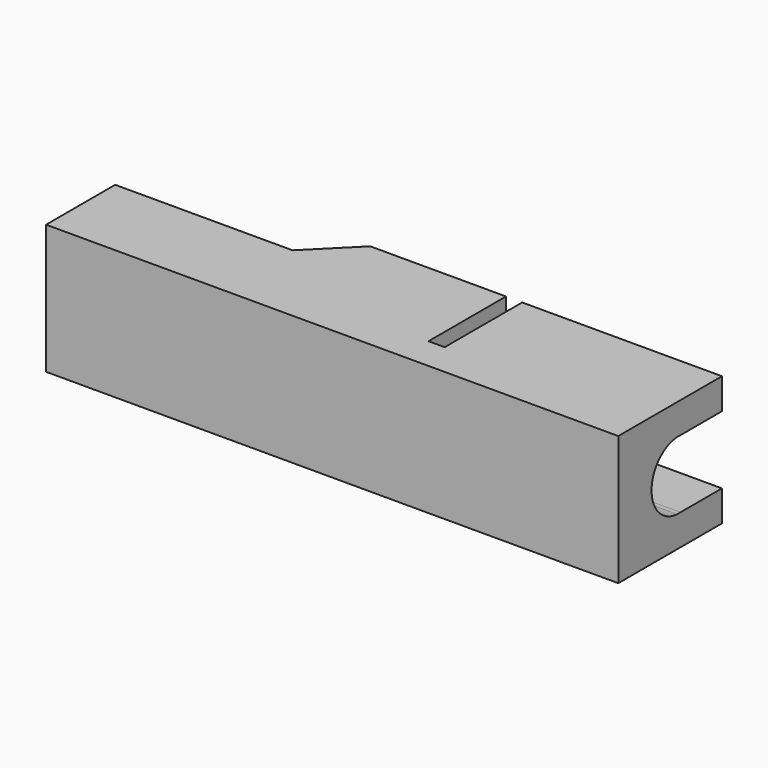
from build123d import *

# Parameters (mm, degrees)
F0_W      = 93
F0_H      = 10
F1_DEPTH  = 12
F3_DEPTH  = 90
F5_W      = 8.9714768017
F5_H      = 12
F6_DEPTH  = 1.5
F7_DEPTH  = 2
F8_DEPTH  = 40
F9_W      = 20.4241964966
F9_H      = 12
F10_DEPTH = 4
F11_SIZE  = 3.99999


# Not quite as in the source:
# - a fillet or chamfer is up to 0.001 mm smaller than in the source, because OpenCascade refuses the exact size


with BuildPart() as f1:
    # F0 (on Top) → F1 (new body)
    with BuildSketch(Plane.XY):
        with Locations((46.5, 5)):
            Rectangle(F0_W, F0_H)
    extrude(amount=F1_DEPTH)

    # F2 (on face) → F3 (cut)
    with BuildSketch(Plane.YZ.offset(93)):
        with BuildLine():
            Line((4.8075824627, 6), (4.8075824627, 9.1441176014))
            ThreePointArc((4.8075824627, 9.1441176014), (1.85, 6), (4.8075824627, 2.8558823986))
            Line((4.8075824627, 2.8558823986), (4.8075824627, 6))
        make_face()
        with BuildLine():
            ThreePointArc((5.1924175373, 9.1441176014), (5, 9.15), (4.8075824627, 9.1441176014))
            Line((4.8075824627, 9.1441176014), (5.1924175373, 9.1441176014))
        make_face()
        with BuildLine():
            Line((5.1924175373, 9.1441176014), (4.8075824627, 9.1441176014))
            Line((4.8075824627, 9.1441176014), (4.8075824627, 6))
            Line((4.8075824627, 6), (8.15, 6))
            ThreePointArc((8.15, 6), (7.2944079021, 8.1582845917), (5.1924175373, 9.1441176014))
        make_face()
        with BuildLine():
            Line((5.1924175373, 2.8558823986), (4.8075824627, 2.8558823986))
            ThreePointArc((4.8075824627, 2.8558823986), (5, 2.85), (5.1924175373, 2.8558823986))
        make_face()
        with BuildLine():
            Line((4.8075824627, 6), (4.8075824627, 2.8558823986))
            Line((4.8075824627, 2.8558823986), (5.1924175373, 2.8558823986))
            ThreePointArc((5.1924175373, 2.8558823986), (7.2944079021, 3.8417154083), (8.15, 6))
            Line((8.15, 6), (4.8075824627, 6))
        make_face()
        with BuildLine():
            Line((10, 9.1441176014), (5.1924175373, 9.1441176014))
            ThreePointArc((5.1924175373, 9.1441176014), (7.2944079021, 8.1582845917), (8.15, 6))
            Line((8.15, 6), (10, 6))
            Line((10, 6), (10, 9.1441176014))
        make_face()
        with BuildLine():
            ThreePointArc((8.15, 6), (7.2944079021, 3.8417154083), (5.1924175373, 2.8558823986))
            Line((5.1924175373, 2.8558823986), (10, 2.8558823986))
            Line((10, 2.8558823986), (10, 6))
            Line((10, 6), (8.15, 6))
        make_face()
    extrude(amount=-F3_DEPTH, mode=Mode.SUBTRACT)

    # F5 (on offset) → F6 (cut)
    with BuildSketch(Plane.YZ.offset(33)):
        with Locations((5.5142615992, 6)):
            Rectangle(F5_W, F5_H)
    extrude(amount=F6_DEPTH, mode=Mode.SUBTRACT)

    # F7 (add): a face of the model
    f7_faces = [f1.faces().sort_by_distance(p)[0] for p in [
        (46.5, 0, 6),
    ]]
    extrude(f7_faces, amount=F7_DEPTH)

    # F8 (cut): a face of the model
    f8_faces = [f1.faces().sort_by_distance(p)[0] for p in [
        (93, 4, 0.1697056275),
    ]]
    extrude(f8_faces, amount=-F8_DEPTH, mode=Mode.SUBTRACT)

    # F9 (on face) → F10 (cut)
    with BuildSketch(Plane(origin=(0, 10, 0), x_dir=(-1, 0, 0), z_dir=(0, 1, 0))):
        with Locations((-10.2120982483, 6)):
            Rectangle(F9_W, F9_H)
    extrude(amount=-F10_DEPTH, mode=Mode.SUBTRACT)

    # F11 (size 4 in the source; OpenCascade refuses exactly that, so slightly less here)
    f11_edges = [f1.edges().sort_by_distance(p)[0] for p in [
        (20.424196, 6, 1.427941),
        (20.424196, 6, 10.572059),
    ]]
    chamfer(f11_edges, length=F11_SIZE)


solid = f1.part
